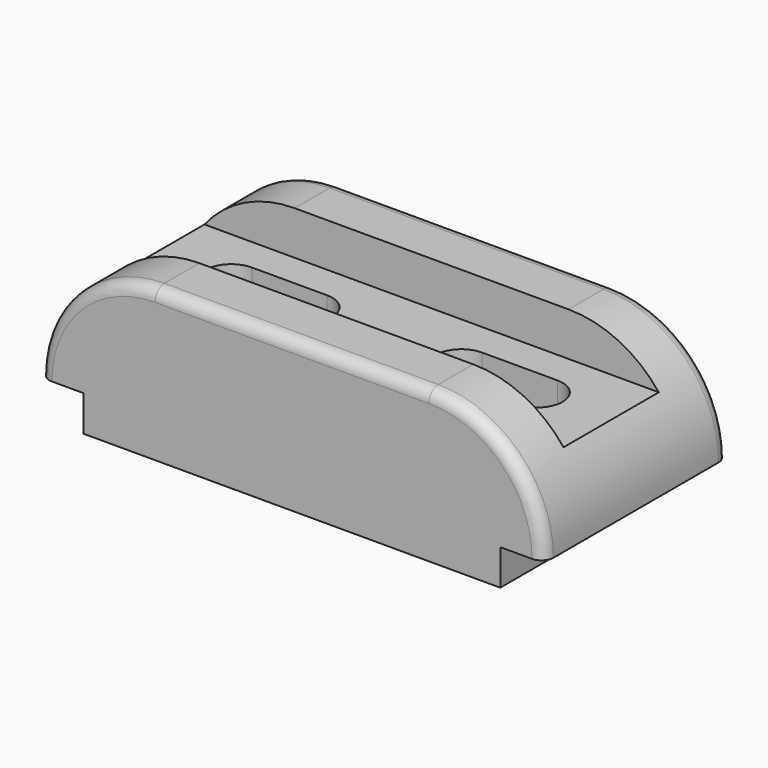
from build123d import *

# Parameters (mm, degrees)
F1_DEPTH      = 29
F2_R          = 3
F3_W          = 30
F3_H          = 11
F4_DEPTH      = 63.5010001
F4_DEPTH_BACK = 63.5010001
F6_DEPTH      = 27.001


with BuildPart() as f1:
    # F0 (on Front) → F1 (new body, symmetric)
    with BuildSketch(Plane.XZ):
        with BuildLine():
            Line((-52.5, 0), (52.5, 0))
            Line((52.5, 0), (52.5, 9))
            Line((52.5, 9), (63.5, 9))
            ThreePointArc((63.5, 9), (55.0060966544, 29.5060966544), (34.5, 38))
            Line((34.5, 38), (-34.5, 38))
            ThreePointArc((-34.5, 38), (-55.0060966544, 29.5060966544), (-63.5, 9))
            Line((-63.5, 9), (-52.5, 9))
            Line((-52.5, 9), (-52.5, 0))
        make_face()
    extrude(amount=F1_DEPTH, both=True)

    # F2
    f2_edges = [f1.edges().sort_by_distance(p)[0] for p in [
        (0, -29, 38),
        (0, 29, 38),
    ]]
    fillet(f2_edges, radius=F2_R)

    # F3 (on Right) → F4 (cut, two sides)
    with BuildSketch(Plane.YZ) as f4_sk:
        with Locations((0, 32.5)):
            Rectangle(F3_W, F3_H)
    extrude(amount=-F4_DEPTH, mode=Mode.SUBTRACT)
    extrude(f4_sk.sketch, amount=F4_DEPTH_BACK, mode=Mode.SUBTRACT)

    # F5 (on face) → F6 (cut, through all)
    with BuildSketch(Plane.XY.offset(27)):
        with BuildLine():
            Line((-19.5, 6.5), (-38.5, 6.5))
            ThreePointArc((-38.5, 6.5), (-45, 0), (-38.5, -6.5))
            Line((-38.5, -6.5), (-19.5, -6.5))
            ThreePointArc((-19.5, -6.5), (-13, 0), (-19.5, 6.5))
        make_face()
        with BuildLine():
            Line((38.5, 6.5), (19.5, 6.5))
            ThreePointArc((19.5, 6.5), (13, 0), (19.5, -6.5))
            Line((19.5, -6.5), (38.5, -6.5))
            ThreePointArc((38.5, -6.5), (45, 0), (38.5, 6.5))
        make_face()
    extrude(amount=-F6_DEPTH, mode=Mode.SUBTRACT)


solid = f1.part
